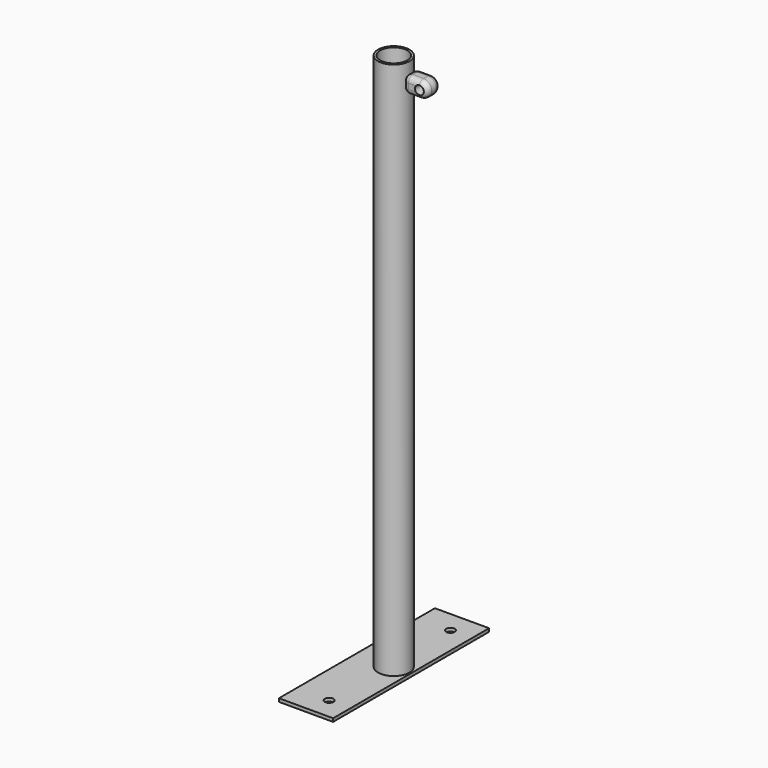
from build123d import *

# Parameters (mm, degrees)
F0_R         = 14.5
F0_R_2       = 12.5
F1_DEPTH     = 500
F2_R         = 4
F2_R_2       = 11
F3_DEPTH     = 3
F4_W         = 15
F4_H         = 15
F5_DEPTH     = 7.5
F6_R         = 5
F7_T1_DEPTH  = 5
F7_T3_DEPTH  = 5
F7_S7_W      = 5
F7_S7_H      = 5
F7_T8_DEPTH  = 5
F7_S13_W     = 5
F7_S13_H     = 5
F7_T14_DEPTH = 5
F7_T18_ANGLE = 90
F7_T20_ANGLE = 90
F9_D         = 8


# Not quite as in the source:
# - a fillet or chamfer that OpenCascade refuses, or shapes differently, is made with other operations: its cross-section is extruded or revolved along the edge and cut away or added


with BuildPart() as f1:
    # F0 (on Top) → F1 (new body)
    with BuildSketch(Plane.XY):
        Circle(F0_R)
        Circle(F0_R_2, mode=Mode.SUBTRACT)
    extrude(amount=F1_DEPTH)

    # F2 (on Top) → F3 (join)
    with BuildSketch(Plane.XY):
        Polygon((16, -90), (16, 0), (16, 90), (-34, 90), (-34, -90), align=None)
        with Locations((-3.6336369812, -70)):
            Circle(F2_R, mode=Mode.SUBTRACT)
        Circle(F2_R_2, mode=Mode.SUBTRACT)
        with Locations((-3.6336369812, 70)):
            Circle(F2_R, mode=Mode.SUBTRACT)
    extrude(amount=F3_DEPTH)


with BuildPart() as f5:
    # F4 (on Front) → F5 (new body, symmetric)
    with BuildSketch(Plane.XZ):
        with Locations((22.0739521831, 484.3088161945)):
            Rectangle(F4_W, F4_H)
        with BuildLine():
            ThreePointArc((29.5739521831, 476.8088161945), (37.0739521831, 484.3088161945), (29.5739521831, 491.8088161945))
            Line((29.5739521831, 491.8088161945), (29.5739521831, 476.8088161945))
        make_face()
    extrude(amount=F5_DEPTH, both=True)

    # F6
    f6_edges = [f5.edges().sort_by_distance(p)[0] for p in [
        (14.573952, -7.5, 484.308816),
        (37.073952, -7.5, 484.308816),
        (22.073952, 7.5, 476.808816),
    ]]
    fillet(f6_edges, radius=F6_R)

    # F7: fillet of radius 5 on 1 edges, made by hand

    # F7_s2 → F7_t1 (cut)
    with BuildSketch(Plane.XY.offset(481.8088161945)):
        with BuildLine():
            ThreePointArc((14.5739521831, 2.5), (16.0384182772, 6.0355339059), (19.5739521831, 7.5))
            Line((19.5739521831, 7.5), (14.5739521831, 7.5))
            Line((14.5739521831, 7.5), (14.5739521831, 2.5))
        make_face()
    extrude(amount=F7_T1_DEPTH, mode=Mode.SUBTRACT)

    # F7_s4 → F7_t3 (cut)
    with BuildSketch(Plane.XZ.offset(-2.5)):
        with BuildLine():
            ThreePointArc((14.5739521831, 481.8088161945), (16.0384182772, 478.2732822886), (19.5739521831, 476.8088161945))
            Line((19.5739521831, 476.8088161945), (14.5739521831, 476.8088161945))
            Line((14.5739521831, 476.8088161945), (14.5739521831, 481.8088161945))
        make_face()
        with BuildLine():
            ThreePointArc((19.5739521831, 491.8088161945), (16.0384182772, 490.3443501005), (14.5739521831, 486.8088161945))
            Line((14.5739521831, 486.8088161945), (14.5739521831, 491.8088161945))
            Line((14.5739521831, 491.8088161945), (19.5739521831, 491.8088161945))
        make_face()
    extrude(amount=F7_T3_DEPTH, mode=Mode.SUBTRACT)


with BuildPart() as f7_tool6:
    # F7_s7 → F7_t8 (new body)
    with BuildSketch(Plane.YZ.offset(19.5739521831)):
        with Locations((-5, 479.3088161945)):
            Rectangle(F7_S7_W, F7_S7_H)
    extrude(amount=-F7_T8_DEPTH)

    # F7_s9 → F7_t10 (revolve, cut)
    with BuildSketch(Plane(origin=(19.5739521831, -2.5, 481.8088161945), x_dir=(0, 0.7071067812, 0.7071067812), z_dir=(0, -0.7071067812, 0.7071067812))):
        with BuildLine():
            ThreePointArc((0, -5), (5, 0), (0, 5))
            Line((0, 5), (0, -5))
        make_face()
    revolve(axis=Axis((19.5739521831, -2.5, 481.8088161945), (-1, 0, 0)), mode=Mode.SUBTRACT)


with BuildPart() as f5_1:
    add(f5.part)

    # F7_t5: cut F7_tool6
    add(f7_tool6.part, mode=Mode.SUBTRACT)


with BuildPart() as f7_tool12:
    # F7_s13 → F7_t14 (new body)
    with BuildSketch(Plane.XY.offset(486.8088161945)):
        with Locations((17.0739521831, -5)):
            Rectangle(F7_S13_W, F7_S13_H)
    extrude(amount=F7_T14_DEPTH)

    # F7_s15 → F7_t16 (revolve, cut)
    with BuildSketch(Plane(origin=(19.5739521831, -2.5, 486.8088161945), x_dir=(0.7071067812, 0.7071067812, 0), z_dir=(0.7071067812, -0.7071067812, 0))):
        with BuildLine():
            ThreePointArc((0, -5), (5, 0), (0, 5))
            Line((0, 5), (0, -5))
        make_face()
    revolve(axis=Axis((19.5739521831, -2.5, 486.8088161945), (0, 0, 1)), mode=Mode.SUBTRACT)


with BuildPart() as f5_2:
    add(f5_1.part)

    # F7_t11: cut F7_tool12
    add(f7_tool12.part, mode=Mode.SUBTRACT)

    # F7_s17 → F7_t18 (revolve, cut)
    with BuildSketch(Plane.XZ.offset(-2.5)):
        with BuildLine():
            ThreePointArc((14.5739521831, 486.8088161945), (16.0384182772, 490.3443501005), (19.5739521831, 491.8088161945))
            Line((19.5739521831, 491.8088161945), (14.5739521831, 491.8088161945))
            Line((14.5739521831, 491.8088161945), (14.5739521831, 486.8088161945))
        make_face()
    revolve(axis=Axis((14.5739521831, 2.5, 486.8088161945), (-1, 0, 0)), revolution_arc=F7_T18_ANGLE, mode=Mode.SUBTRACT)

    # F7_s19 → F7_t20 (revolve, cut)
    with BuildSketch(Plane.XZ.offset(-2.5)):
        with BuildLine():
            ThreePointArc((14.5739521831, 481.8088161945), (16.0384182772, 478.2732822886), (19.5739521831, 476.8088161945))
            Line((19.5739521831, 476.8088161945), (14.5739521831, 476.8088161945))
            Line((14.5739521831, 476.8088161945), (14.5739521831, 481.8088161945))
        make_face()
    revolve(axis=Axis((14.5739521831, 2.5, 481.8088161945), (1, 0, 0)), revolution_arc=F7_T20_ANGLE, mode=Mode.SUBTRACT)

    # F9 (through all)
    with Locations(Plane.XZ.offset(7.5)):
        with Locations((29.5739521831, 484.3088161945)):
            Hole(F9_D / 2)


solid = Compound([f1.part, f5_2.part])
